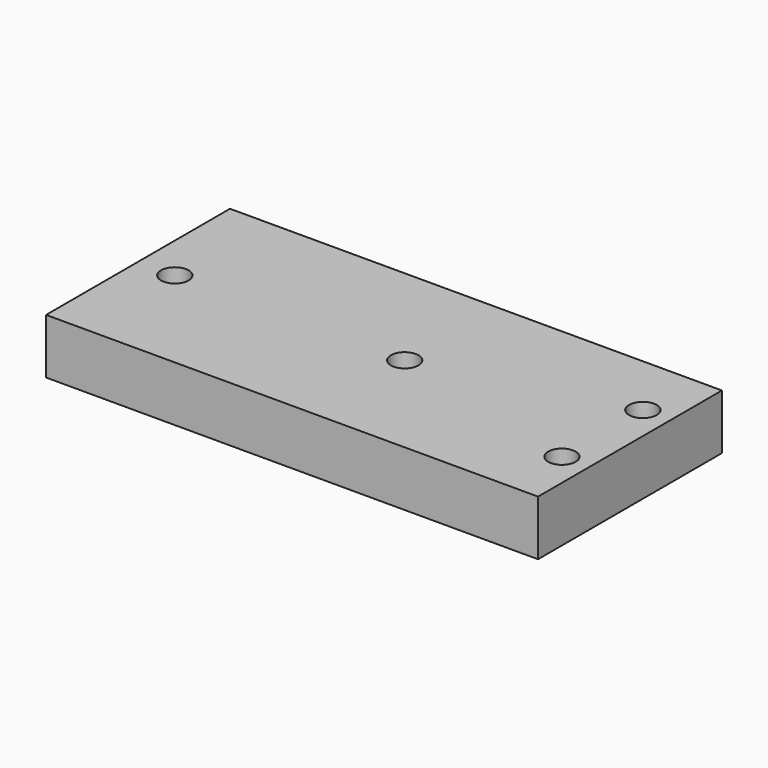
from build123d import *

# Parameters (mm, degrees)
F0_W     = 55
F0_H     = 25
F1_DEPTH = 6
F2_D     = 3
F3_DEPTH = 1.5


# Not quite as in the source:
# - a feature names something its author has since deleted; it is built from what else it names


with BuildPart() as f1:
    # F0 (on Top) → F1 (new body)
    with BuildSketch(Plane.XY):
        Rectangle(F0_W, F0_H)
    extrude(amount=F1_DEPTH)

    # F2 (through all)
    with Locations(Plane(origin=(0, 0, 0), x_dir=(1, 0, 0), z_dir=(0, 0, -1))):
        with Locations((-23.5, 0), (23, -5.5), (23, 5.5), (1.5, 0)):
            Hole(F2_D / 2)

    # F3 (cut): a face of the model
    f3_faces = [f1.faces().sort_by_distance(p)[0] for p in [
        (27.5, 0, 3),
    ]]
    extrude(f3_faces, amount=-F3_DEPTH, mode=Mode.SUBTRACT)


solid = f1.part
